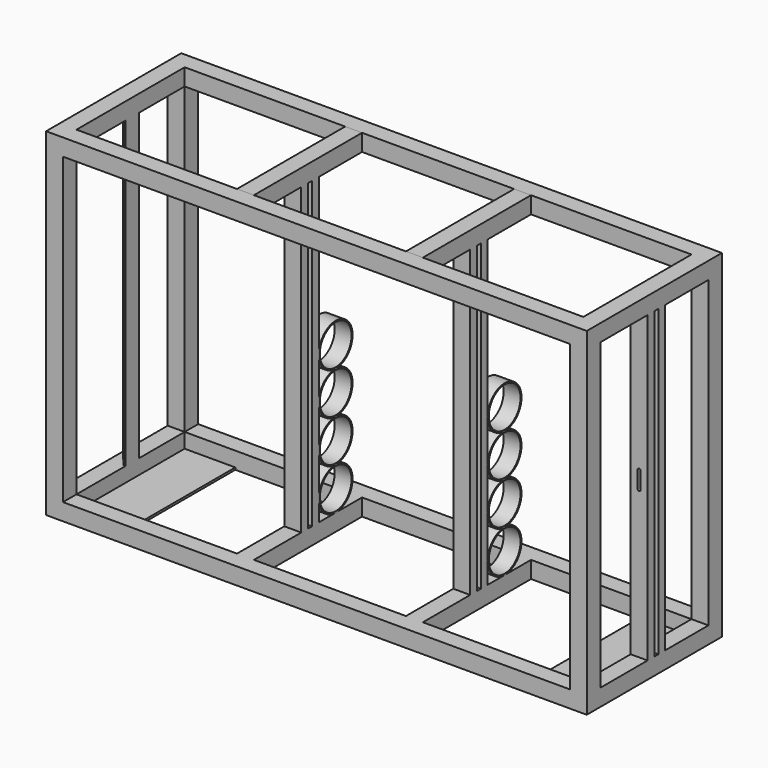
from build123d import *

# Parameters (mm, degrees)
F0_W      = 1280
F0_H      = 400
F1_DEPTH  = 800
F2_W      = 1200
F2_H      = 320
F3_DEPTH  = 800.001
F4_W      = 1200
F4_H      = 720
F5_DEPTH  = 400.001
F6_W      = 320
F6_H      = 720
F7_DEPTH  = 1280.001
F8_W      = 40
F8_H      = 40
F9_DEPTH  = 320
F10_W     = 40
F10_H     = 40
F11_DEPTH = 320
F12_W     = 40
F12_H     = 20
F12_W_2   = 15.5
F12_H_2   = 4.5
F14_R     = 47
F15_DEPTH = 440
F16_W     = 360
F16_H     = 430
F17_DEPTH = 220.001
F18_W     = 120
F18_H     = 5
F19_DEPTH = 320
F20_W     = 40
F20_H     = 20
F21_DEPTH = 720
F23_DEPTH = 52


with BuildPart() as f1:
    # F0 (on Top) → F1 (new body)
    with BuildSketch(Plane.XY):
        with Locations((640, 200)):
            Rectangle(F0_W, F0_H)
    extrude(amount=F1_DEPTH)

    # F2 (on face) → F3 (cut, through all)
    with BuildSketch(Plane.XY.offset(800)):
        with Locations((640, 200)):
            Rectangle(F2_W, F2_H)
    extrude(amount=-F3_DEPTH, mode=Mode.SUBTRACT)

    # F4 (on face) → F5 (cut, through all)
    with BuildSketch(Plane.XZ):
        with Locations((640, 400)):
            Rectangle(F4_W, F4_H)
    extrude(amount=-F5_DEPTH, mode=Mode.SUBTRACT)

    # F6 (on face) → F7 (cut, through all)
    with BuildSketch(Plane.YZ.offset(1280)):
        with Locations((200, 400)):
            Rectangle(F6_W, F6_H)
    extrude(amount=-F7_DEPTH, mode=Mode.SUBTRACT)

    # F8 (on face) → F9 (join, through all)
    with BuildSketch(Plane.XZ.offset(-360)):
        with Locations((440, 20)):
            Rectangle(F8_W, F8_H)
        with Locations((840, 20)):
            Rectangle(F8_W, F8_H)
    extrude(amount=F9_DEPTH)

    # F10 (on face) → F11 (join, through all)
    with BuildSketch(Plane.XZ.offset(-360)):
        with Locations((440, 779.9999904633)):
            Rectangle(F10_W, F10_H)
        with Locations((840, 779.9999904633)):
            Rectangle(F10_W, F10_H)
    extrude(amount=F11_DEPTH)

    # F12 (on face) → F13 (join, up to the next surface of F1)
    with BuildSketch(Plane.XY.offset(40)):
        with Locations((440, 190)):
            Rectangle(F12_W, F12_H)
        with Locations((840, 222)):
            Rectangle(F12_W, F12_H)
        with Locations((840, 190)):
            Rectangle(F12_W, F12_H)
        with Locations((440, 222)):
            Rectangle(F12_W, F12_H)
        with Locations((27.75, 205)):
            Rectangle(F12_W_2, F12_H_2)
        Polygon((40, 185), (40, 225), (35.5, 225), (35.5, 207.25), (35.5, 202.75), (35.5, 185), align=None)
    extrude(until=Until.NEXT)



with BuildPart() as f15:
    # F14 (on face) → F15 (new body)
    with BuildSketch(Plane.YZ.offset(860)):
        with BuildLine():
            ThreePointArc((232.0000026226, 390), (246.6446635633, 354.6446609407), (282.0000026227, 340))
            ThreePointArc((282.0000026227, 340), (317.355341682, 354.6446609407), (332.0000026226, 390))
            ThreePointArc((332.0000026226, 390), (282.0000026226, 440), (232.0000026226, 390))
        make_face()
        with Locations((282.0000026226, 390)):
            Circle(F14_R, mode=Mode.SUBTRACT)
    extrude(amount=-F15_DEPTH)

    # F14 (on face) → F15, piece 2 (join)
    with BuildSketch(Plane.YZ.offset(860)):
        with BuildLine():
            ThreePointArc((232.0000026226, 290), (246.6446630019, 254.6446615021), (282.0000010347, 240))
            ThreePointArc((282.0000010347, 240), (317.3553411205, 254.6446603792), (332.0000026226, 290))
            ThreePointArc((332.0000026226, 290), (317.355341682, 325.3553390593), (282.0000026227, 340))
            ThreePointArc((282.0000026227, 340), (246.6446635633, 325.3553390593), (232.0000026226, 290))
        make_face()
        with Locations((282.0000026226, 290)):
            Circle(F14_R, mode=Mode.SUBTRACT)
    extrude(amount=-F15_DEPTH)


with BuildPart() as f1_1:
    add(f1.part)

    add(f15.part)  # F15#3 merges F15
    # F14 (on face) → F15, piece 3 (join)
    with BuildSketch(Plane.YZ.offset(860)):
        with BuildLine():
            ThreePointArc((232, 189.9999997472), (246.6446610932, 154.6446607881), (282.0000001788, 140))
            ThreePointArc((282.0000001788, 140), (317.3553391225, 154.6446610039), (332, 190))
            ThreePointArc((332, 190), (317.3553394251, 225.3553386935), (282.0000010347, 240))
            ThreePointArc((282.0000010347, 240), (246.6446612171, 225.3553393358), (232, 189.9999997472))
        make_face()
        with Locations((282, 190)):
            Circle(F14_R, mode=Mode.SUBTRACT)
        with BuildLine():
            ThreePointArc((282, 40), (317.3553390593, 54.6446609407), (332, 90))
            ThreePointArc((332, 90), (317.3553391225, 125.3553389961), (282.0000001788, 140))
            ThreePointArc((282.0000001788, 140), (246.6446610039, 125.3553391225), (232, 90))
            ThreePointArc((232, 90), (246.6446609407, 54.6446609407), (282, 40))
        make_face()
        with Locations((282, 90)):
            Circle(F14_R, mode=Mode.SUBTRACT)
    extrude(amount=-F15_DEPTH)

    # F16 (on face) → F17 (cut, through all)
    with BuildSketch(Plane.XZ.offset(-180)):
        with Locations((640, 255)):
            Rectangle(F16_W, F16_H)
    extrude(amount=-F17_DEPTH, mode=Mode.SUBTRACT)

    # F18 (on face) → F19 (join, through all)
    with BuildSketch(Plane.XZ.offset(-360)):
        with Locations((100, 2.5)):
            Rectangle(F18_W, F18_H)
        with Locations((1180, 2.5)):
            Rectangle(F18_W, F18_H)
    extrude(amount=F19_DEPTH)

    # F20 (on face) → F21 (join, through all)
    with BuildSketch(Plane.XY.offset(40)):
        with Locations((1260, 190)):
            Rectangle(F20_W, F20_H)
        with Locations((1260, 222)):
            Rectangle(F20_W, F20_H)
    extrude(amount=F21_DEPTH)

    # F22 (on face) → F23 (cut, through all)
    with BuildSketch(Plane.XZ.offset(-180)):
        with BuildLine():
            Line((1256.5, 430), (1256.5, 390))
            ThreePointArc((1256.5, 390), (1260, 386.5), (1263.5, 390))
            Line((1263.5, 390), (1263.5, 430))
            ThreePointArc((1263.5, 430), (1260, 433.5), (1256.5, 430))
        make_face()
    extrude(amount=-F23_DEPTH, mode=Mode.SUBTRACT)


solid = f1_1.part
